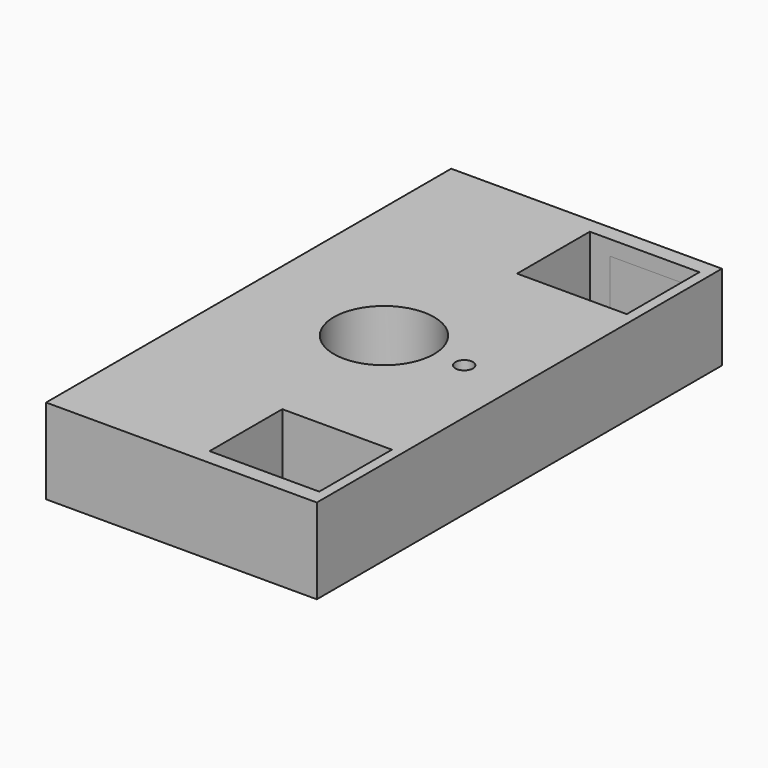
from build123d import *

# Parameters (mm, degrees)
F0_R      = 10
F0_W      = 21.869414486
F0_H      = 18.1213598698
F1_DEPTH  = 17
F3_DEPTH  = 15
F4_W      = 7
F4_H      = 3
F5_DEPTH  = 5
F7_DEPTH  = 14
F8_SIZE   = 2
F9_W      = 18
F9_H      = 6
F10_DEPTH = 6


# Not quite as in the source:
# - a feature names something its author has since deleted; it is built from what else it names


with BuildPart() as f1:
    # F0 (on Top) → F1 (new body)
    with BuildSketch(Plane.XY):
        Polygon((27, -38.3339710534), (27, 50.5), (-27, 50.5), (-27, -50.5), (27, -50.5), align=None)
        Polygon((25, -29.2732911184), (25, -38.3339710534), (25, -47.3946509883), (3.130585514, -47.3946509883), (3.130585514, -29.2732911184), align=None, mode=Mode.SUBTRACT)
        Circle(F0_R, mode=Mode.SUBTRACT)
        with BuildLine():
            ThreePointArc((17.75, 0), (16, -1.75), (14.25, 0))
            ThreePointArc((14.25, 0), (16, 1.75), (17.75, 0))
        make_face(mode=Mode.SUBTRACT)
        with Locations((14.065292757, 38.3339710534)):
            Rectangle(F0_W, F0_H, mode=Mode.SUBTRACT)
    extrude(amount=F1_DEPTH)

    # F2 (on face) → F3 (cut)
    with BuildSketch(Plane(origin=(0, 0, 0), x_dir=(1, 0, 0), z_dir=(0, 0, -1))):
        Polygon((7.125, 26), (7.125, 0), (7.125, -26), (24.875, -26), (24.875, 23), (17.875, 23), (17.875, 26), align=None)
        with BuildLine():
            ThreePointArc((20.5, 0), (16, -4.5), (11.5, 0))
            ThreePointArc((11.5, 0), (16, 4.5), (20.5, 0))
        make_face(mode=Mode.SUBTRACT)
        with BuildLine():
            Line((-11.8641304348, -45), (-11.8641304348, 0))
            Line((-11.8641304348, 0), (-11.8641304348, 45))
            Line((-11.8641304348, 45), (-14.3641304348, 45))
            Line((-14.3641304348, 45), (-14.3641304348, 46))
            Line((-14.3641304348, 46), (-11.8431356333, 46))
            Line((-11.8431356333, 46), (-11.8431356333, 47))
            Line((-11.8431356333, 47), (-14.3641304348, 47))
            ThreePointArc((-14.3641304348, 47), (-17, 49.6358695652), (-19.6358695652, 47))
            Line((-19.6358695652, 47), (-22.1358695652, 47))
            Line((-22.1358695652, 47), (-22.1358695652, 46))
            Line((-22.1358695652, 46), (-19.6358695652, 46))
            Line((-19.6358695652, 46), (-19.6358695652, 45))
            Line((-19.6358695652, 45), (-22.1358695652, 45))
            Line((-22.1358695652, 45), (-22.1358695652, -45))
            Line((-22.1358695652, -45), (-19.6358695652, -45))
            Line((-19.6358695652, -45), (-19.6358695652, -46))
            Line((-19.6358695652, -46), (-22.1358695652, -46))
            Line((-22.1358695652, -46), (-22.1358695652, -47))
            Line((-22.1358695652, -47), (-19.6358695652, -47))
            ThreePointArc((-19.6358695652, -47), (-17, -49.6358695652), (-14.3641304348, -47))
            Line((-14.3641304348, -47), (-11.8431356333, -47))
            Line((-11.8431356333, -47), (-11.8431356333, -46))
            Line((-11.8431356333, -46), (-14.3641304348, -46))
            Line((-14.3641304348, -46), (-14.3641304348, -45))
            Line((-14.3641304348, -45), (-11.8641304348, -45))
        make_face()
    extrude(amount=-F3_DEPTH, mode=Mode.SUBTRACT)

    # F4 (on face) → F5 (cut)
    with BuildSketch(Plane(origin=(0, 0, 0), x_dir=(1, 0, 0), z_dir=(0, 0, -1))):
        with Locations((21.5, 24.5)):
            Rectangle(F4_W, F4_H)
        with BuildLine():
            Line((0, 29.1349645704), (0, 39.6236035006))
            ThreePointArc((0, 39.6236035006), (-2.9289321881, 46.6946713125), (-10, 49.6236035006))
            Line((-10, 49.6236035006), (-17, 49.6358695652))
            Line((-17, 49.6358695652), (-17, 47.6358695652))
            Line((-17, 47.6358695652), (-10, 47.6358695652))
            ThreePointArc((-10, 47.6358695652), (-4.3388107028, 45.2883854424), (-2.0000094035, 39.6236035006))
            Line((-2.0000094035, 39.6236035006), (-2.0000094035, 29.1349645704))
            ThreePointArc((-2.0000094035, 29.1349645704), (0.5848933582, 22.5223852264), (7.1590254083, 19.8412071913))
            Line((7.1590254083, 19.8412071913), (7.125, 21.6599348028))
            ThreePointArc((7.125, 21.6599348028), (1.9168065811, 23.8288183935), (0, 29.1349645704))
        make_face()
        with BuildLine():
            ThreePointArc((7.1590254083, -19.8412071913), (0.5848933582, -22.5223852264), (-2.0000094035, -29.1349645704))
            Line((-2.0000094035, -29.1349645704), (-2.0000094035, -39.6236035006))
            ThreePointArc((-2.0000094035, -39.6236035006), (-4.3388107028, -45.2883854424), (-10, -47.6358695652))
            Line((-10, -47.6358695652), (-17, -47.6358695652))
            Line((-17, -47.6358695652), (-17, -49.6358695652))
            Line((-17, -49.6358695652), (-10, -49.6236035006))
            ThreePointArc((-10, -49.6236035006), (-2.9289321881, -46.6946713125), (0, -39.6236035006))
            Line((0, -39.6236035006), (0, -29.1349645704))
            ThreePointArc((0, -29.1349645704), (1.9168065811, -23.8288183935), (7.125, -21.6599348028))
            Line((7.125, -21.6599348028), (7.1590254083, -19.8412071913))
        make_face()
    extrude(amount=-F5_DEPTH, mode=Mode.SUBTRACT)

    # F6 (on face) → F7 (cut)
    with BuildSketch(Plane(origin=(0, 0, 0), x_dir=(1, 0, 0), z_dir=(0, 0, -1))):
        with BuildLine():
            ThreePointArc((24.25, 24.75), (23.5, 25.5), (22.75, 24.75))
            ThreePointArc((22.75, 24.75), (23.5, 24), (24.25, 24.75))
        make_face()
        Polygon((7.125, -26), (7.125, -36.75), (7.125, -47.5), (24.875, -47.5), (24.875, -26), align=None)
    extrude(amount=-F7_DEPTH, mode=Mode.SUBTRACT)

    # F8
    f8_edges = [f1.edges().sort_by_distance(p)[0] for p in [
        (14.25, 0, 0),
    ]]
    chamfer(f8_edges, length=F8_SIZE)

    # F9 (on face) → F10 (join)
    with BuildSketch(Plane.XY.offset(17)):
        with Locations((16.0392038773, 22.9714149609)):
            Rectangle(F9_W, F9_H)
    extrude(amount=-F10_DEPTH)


solid = f1.part
